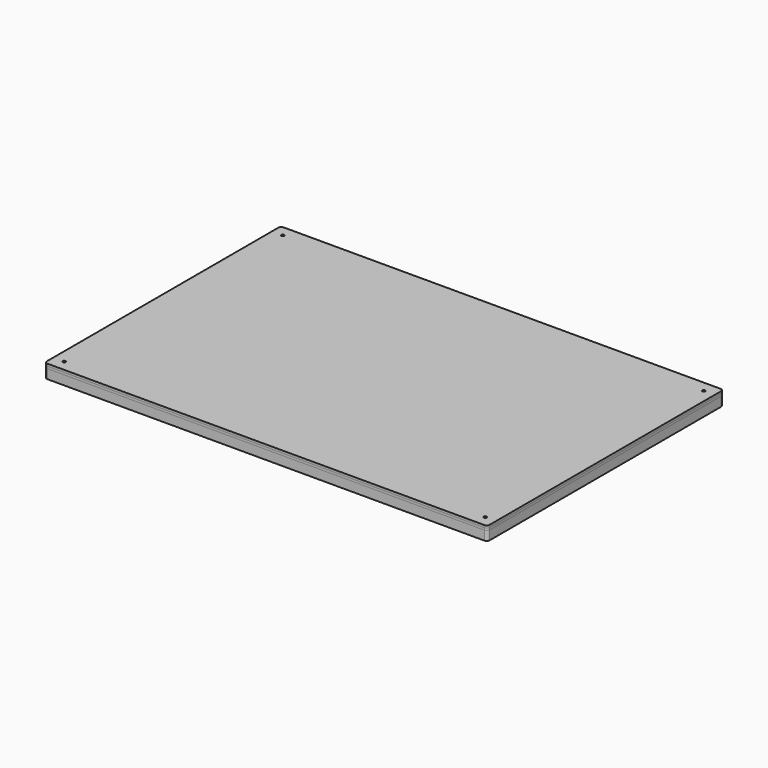
from build123d import *

# Parameters (mm, degrees)
F0_W     = 609.6
F0_H     = 406.4
F0_R     = 2
F0_R_2   = 3.95
F1_DEPTH = 12.7
F2_W     = 609.6
F2_H     = 406.4
F2_R     = 2
F3_DEPTH = 3
F4_R     = 4
F4_2_R   = 4
F5_R     = 2
F6_DEPTH = 3.175


# Not quite as in the source:
# - a length typed as a fraction of an inch, garbled in the dataset ("3 / 203.2 mm" for 3/8 in), is restored


with BuildPart() as f1:
    # F0 (on Top) → F1 (new body)
    with BuildSketch(Plane.XY):
        Rectangle(F0_W, F0_H)
        with Locations((-297.8, -196.2)):
            Circle(F0_R, mode=Mode.SUBTRACT)
        with Locations((-289.7999969482, -188.1999969482)):
            Circle(F0_R_2, mode=Mode.SUBTRACT)
        with Locations((0, -196.2)):
            Circle(F0_R, mode=Mode.SUBTRACT)
        with Locations((297.8, -196.2)):
            Circle(F0_R, mode=Mode.SUBTRACT)
        with Locations((289.7999969482, -188.1999969482)):
            Circle(F0_R_2, mode=Mode.SUBTRACT)
        with Locations((-289.7999969482, 188.1999969482)):
            Circle(F0_R_2, mode=Mode.SUBTRACT)
        with Locations((-297.8, 196.2)):
            Circle(F0_R, mode=Mode.SUBTRACT)
        with Locations((0, 196.2)):
            Circle(F0_R, mode=Mode.SUBTRACT)
        with Locations((289.7999969482, 188.1999969482)):
            Circle(F0_R_2, mode=Mode.SUBTRACT)
        with Locations((297.8, 196.2)):
            Circle(F0_R, mode=Mode.SUBTRACT)
    extrude(amount=F1_DEPTH)

    # F4
    f4_edges = [f1.edges().sort_by_distance(p)[0] for p in [
        (-304.8, -203.2, 6.35),
        (-304.8, 203.2, 6.35),
        (304.8, -203.2, 6.35),
        (304.8, 203.2, 6.35),
    ]]
    fillet(f4_edges, radius=F4_R)


with BuildPart() as f3:
    # F2 (on face) → F3 (new body)
    with BuildSketch(Plane.XY.offset(12.7)):
        Rectangle(F2_W, F2_H)
        with Locations((-297.8, -196.2)):
            Circle(F2_R, mode=Mode.SUBTRACT)
        with Locations((-289.7999969482, -188.1999969482)):
            Circle(F2_R, mode=Mode.SUBTRACT)
        with Locations((0, -196.2)):
            Circle(F2_R, mode=Mode.SUBTRACT)
        with Locations((297.8, -196.2)):
            Circle(F2_R, mode=Mode.SUBTRACT)
        with Locations((289.7999969482, -188.1999969482)):
            Circle(F2_R, mode=Mode.SUBTRACT)
        with Locations((-289.7999969482, 188.1999969482)):
            Circle(F2_R, mode=Mode.SUBTRACT)
        with Locations((-297.8, 196.2)):
            Circle(F2_R, mode=Mode.SUBTRACT)
        with Locations((0, 196.2)):
            Circle(F2_R, mode=Mode.SUBTRACT)
        with Locations((289.7999969482, 188.1999969482)):
            Circle(F2_R, mode=Mode.SUBTRACT)
        with Locations((297.8, 196.2)):
            Circle(F2_R, mode=Mode.SUBTRACT)
    extrude(amount=F3_DEPTH)

    # F4#2
    f4_2_edges = [f3.edges().sort_by_distance(p)[0] for p in [
        (-304.8, -203.2, 14.2),
        (-304.8, 203.2, 14.2),
        (304.8, -203.2, 14.2),
        (304.8, 203.2, 14.2),
    ]]
    fillet(f4_2_edges, radius=F4_2_R)


with BuildPart() as f6:
    # F5 (on face) → F6 (new body)
    with BuildSketch(Plane.XY.offset(15.7)):
        with BuildLine():
            Line((-300.8, -203.2), (300.8, -203.2))
            ThreePointArc((300.8, -203.2), (303.6284271247, -202.0284271247), (304.8, -199.2))
            Line((304.8, -199.2), (304.8, 199.2))
            ThreePointArc((304.8, 199.2), (303.6284271247, 202.0284271247), (300.8, 203.2))
            Line((300.8, 203.2), (-300.8, 203.2))
            ThreePointArc((-300.8, 203.2), (-303.6284271247, 202.0284271247), (-304.8, 199.2))
            Line((-304.8, 199.2), (-304.8, -199.2))
            ThreePointArc((-304.8, -199.2), (-303.6284271247, -202.0284271247), (-300.8, -203.2))
        make_face()
        with Locations((-289.7999969482, -188.1999969482)):
            Circle(F5_R, mode=Mode.SUBTRACT)
        with Locations((289.7999969482, -188.1999969482)):
            Circle(F5_R, mode=Mode.SUBTRACT)
        with Locations((-289.7999969482, 188.1999969482)):
            Circle(F5_R, mode=Mode.SUBTRACT)
        with Locations((289.7999969482, 188.1999969482)):
            Circle(F5_R, mode=Mode.SUBTRACT)
    extrude(amount=F6_DEPTH)


solid = Compound([f1.part, f3.part, f6.part])
